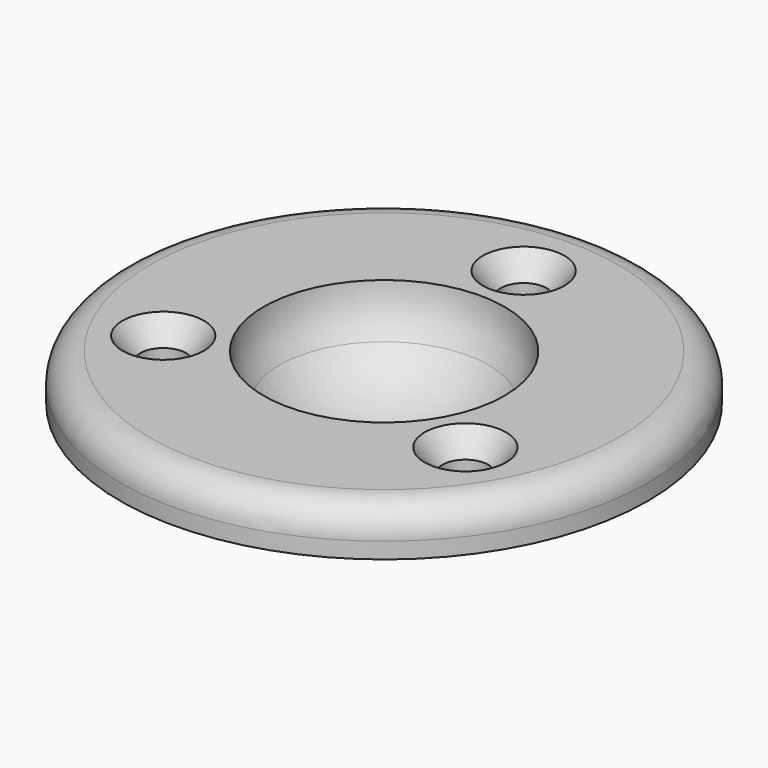
from build123d import *

# Parameters (mm, degrees)
F3_R            = 3.302
F5_D            = 5.08
F5_CSINK_D      = 9.017
F5_CSINK_ANGLE  = 76
F5_COPIES_COUNT = 3
F7_D            = 0.762


# Not quite as in the source:
# - a pattern or mirror of a feature is missing from the dataset's text; its kind, count and spacing are read off the source's solid


with BuildPart() as f2:
    # F1 (on Front) → F2 (revolve)
    with BuildSketch(Plane.XZ):
        with BuildLine():
            add(Edge.make_bspline(
                [(0, -10.16), (7.6989658396, -10.16), (11.5484487595, -5.08)],
                knots=[1.5707963268, 1.5707963268, 1.5707963268, 2.617993878, 2.617993878, 2.617993878], degree=2, weights=[1, 0.8660254038, 1]))
            Line((0, -10.16), (0, -12.7))
            add(Edge.make_bspline(
                [(0, -12.7), (10.3926270225, -12.7), (14.5496778315, -5.08)],
                knots=[1.5707963268, 1.5707963268, 1.5707963268, 2.7300758075, 2.7300758075, 2.7300758075], degree=2, weights=[1, 0.8366600265, 1]))
            Line((14.5496778315, -5.08), (11.5484487595, -5.08))
        make_face()
        with BuildLine():
            Line((29.21, 0), (15.875, 0))
            add(Edge.make_bspline(
                [(14.5496778315, -5.08), (15.875, -2.650644337), (15.875, 0)],
                knots=[2.7300758075, 2.7300758075, 2.7300758075, 3.1415926536, 3.1415926536, 3.1415926536], degree=2, weights=[1, 0.9789063129, 1]))
            Line((14.5496778315, -5.08), (29.21, -5.08))
            Line((29.21, -5.08), (29.21, 0))
        make_face()
        with BuildLine():
            Line((15.875, 0), (13.335, 0))
            add(Edge.make_bspline(
                [(11.5484487595, -5.08), (13.335, -2.7223637951), (13.335, 0)],
                knots=[2.617993878, 2.617993878, 2.617993878, 3.1415926536, 3.1415926536, 3.1415926536], degree=2, weights=[1, 0.9659258263, 1]))
            Line((11.5484487595, -5.08), (14.5496778315, -5.08))
            add(Edge.make_bspline(
                [(14.5496778315, -5.08), (15.875, -2.650644337), (15.875, 0)],
                knots=[2.7300758075, 2.7300758075, 2.7300758075, 3.1415926536, 3.1415926536, 3.1415926536], degree=2, weights=[1, 0.9789063129, 1]))
        make_face()
    revolve(axis=Axis((0, 0, -2.54), (0, 0, -1)))

    # F3
    f3_edges = [f2.edges().sort_by_distance(p)[0] for p in [
        (-29.21, 0, 0),
    ]]
    fillet(f3_edges, radius=F3_R)

    # F5 (through all)
    with Locations(Plane.XY):
        with Locations((0, 19.304)):
            f5 = CounterSinkHole(F5_D / 2, F5_CSINK_D / 2, counter_sink_angle=F5_CSINK_ANGLE)

    # F5_copies: F5 ×3 about axis
    f5_copies_axis = Axis((0, 0, 0), (0, 0, 1))
    for i in range(1, F5_COPIES_COUNT):
        add(f5.rotate(f5_copies_axis, i * 360 / F5_COPIES_COUNT), mode=Mode.SUBTRACT)

    # F7 (through all)
    with Locations(Plane.XY):
        with Locations((-0.635, 0)):
            f7 = Hole(F7_D / 2)

    # F7_copies: F7 across plane
    add(f7.mirror(Plane(origin=(1e-06, 0, 0), x_dir=(0, 0, 1), z_dir=(1, 0, 0))), mode=Mode.SUBTRACT)


solid = f2.part
